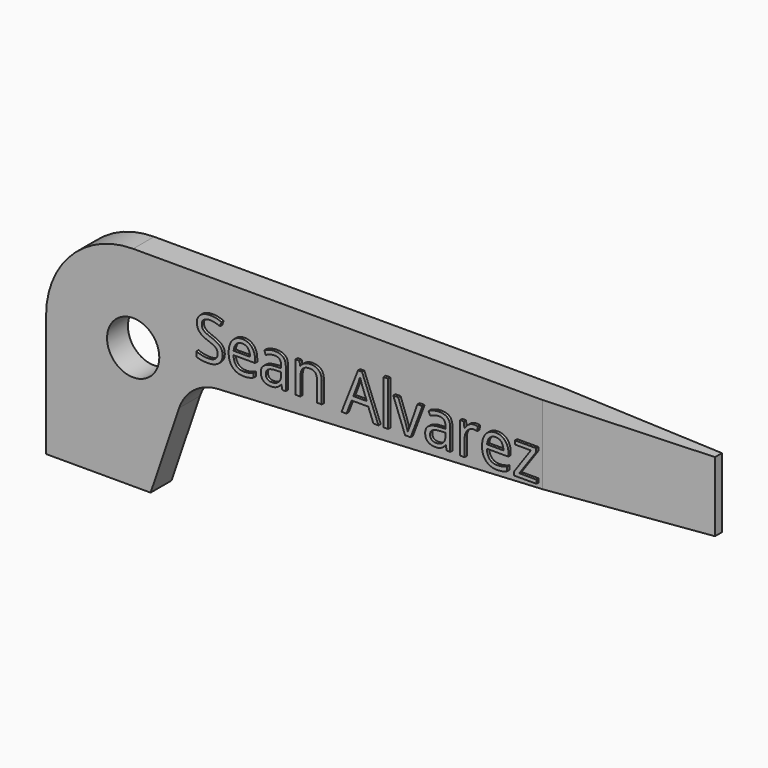
from build123d import *

# Parameters (mm, degrees)
F1_DEPTH     = 2.38125
F2_R         = 2.38125
F3_DEPTH     = 2.38225
F5_DEPTH     = 25.4
F6_TEXT_SIZE = 5.3189023228
F7_DEPTH     = 0.254


# Not quite as in the source:
# - Text() gives the source's letters only with a copy of the font that has no kerning and outlines rounded to 1/6400 em; it was checked with that copy


with BuildPart() as f1:
    # F0 (on Front) → F1 (new body)
    with BuildSketch(Plane.XZ):
        with BuildLine():
            Line((60.325, 19.05), (7.9375, 19.05))
            ThreePointArc((7.9375, 19.05), (2.3248399243, 16.7251600757), (0, 11.1125))
            Line((0, 11.1125), (0, 0))
            Line((0, 0), (9.525, 0))
            Line((9.525, 0), (12.1173647876, 7.6271664624))
            ThreePointArc((12.1173647876, 7.6271664624), (13.4786145605, 9.5135918491), (15.6631963617, 10.3130942181))
            Line((15.6631963617, 10.3130942181), (60.325, 12.7))
            Line((60.325, 12.7), (60.325, 19.05))
        make_face()
    extrude(amount=F1_DEPTH)

    # F2 (on face) → F3 (cut, through all)
    with BuildSketch(Plane.XZ.offset(2.38125)):
        with Locations((7.9375, 11.1125)):
            Circle(F2_R)
    extrude(amount=-F3_DEPTH, mode=Mode.SUBTRACT)

    # F4 (on face) → F5 (cut)
    with BuildSketch(Plane.XY.offset(19.05)):
        Polygon((60.325, -2.38125), (60.325, -1.5875), (45.24375, -2.38125), align=None)
        Polygon((60.325, 0), (45.24375, 0), (60.325, -0.79375), align=None)
    extrude(amount=-F5_DEPTH, mode=Mode.SUBTRACT)

    # F6 (on face) → F7 (join)
    with BuildSketch(Plane.XZ.offset(2.38125)):
        with Locations((13.6228756911, 12.3170241714)):
            Text('Sean Alvarez', F6_TEXT_SIZE, font='Open Sans', text_align=(TextAlign.LEFT, TextAlign.BOTTOM))
    extrude(amount=F7_DEPTH)


solid = f1.part
